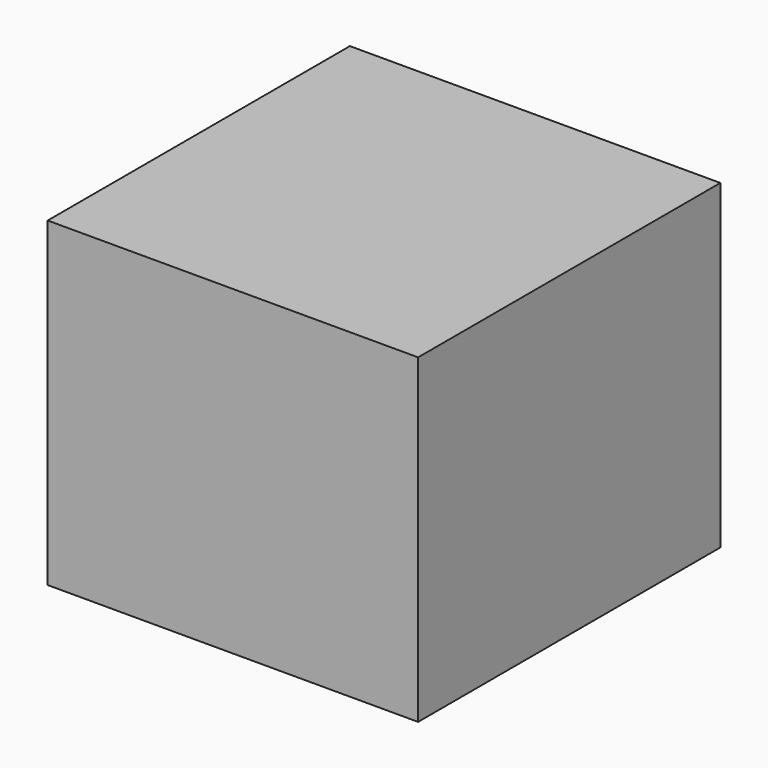
from build123d import *

# Parameters (mm, degrees)
F1_DEPTH = 50.9690083563


# Not quite as in the source:
# - the program builds the solid bodies; features that only make, move or delete a surface that nothing else refers to are left out


with BuildPart() as f1:
    # F0 (on Front) → F1 (new body)
    with BuildSketch(Plane.XZ):
        Polygon((49.9831289053, 0), (0, 0), (0, -43.306723237), (49.9831289053, -43.306723237), (49.9831289053, -21.6533616185), (49.9831289053, -6.6764801741), align=None)
    extrude(amount=-F1_DEPTH)


solid = f1.part
